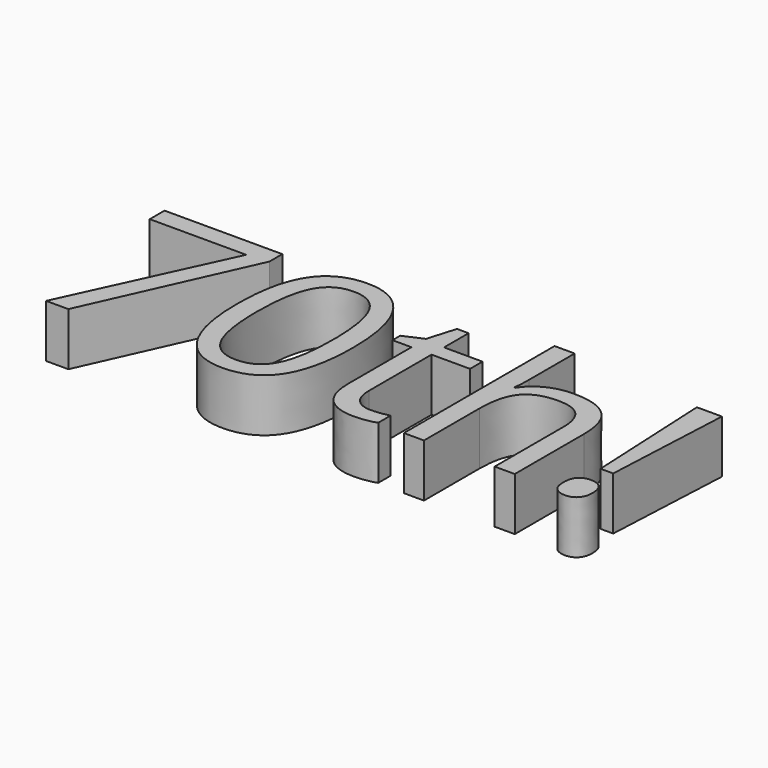
from build123d import *

# Parameters (mm, degrees)
F0_TEXT_SIZE = 23.4127620287
F1_DEPTH     = 5


# Not quite as in the source:
# - Text() gives the source's letters only with a copy of the font that has no kerning and outlines rounded to 1/6400 em; it was checked with that copy


with BuildPart() as f1:
    # F0 (on Top) → F1 (new body)
    with BuildSketch(Plane.XY):
        with Locations((-7.4311275966, -10.5731477961)):
            Text('70th!', F0_TEXT_SIZE, font='Open Sans', text_align=(TextAlign.LEFT, TextAlign.BOTTOM))
    extrude(amount=F1_DEPTH)


solid = f1.part
